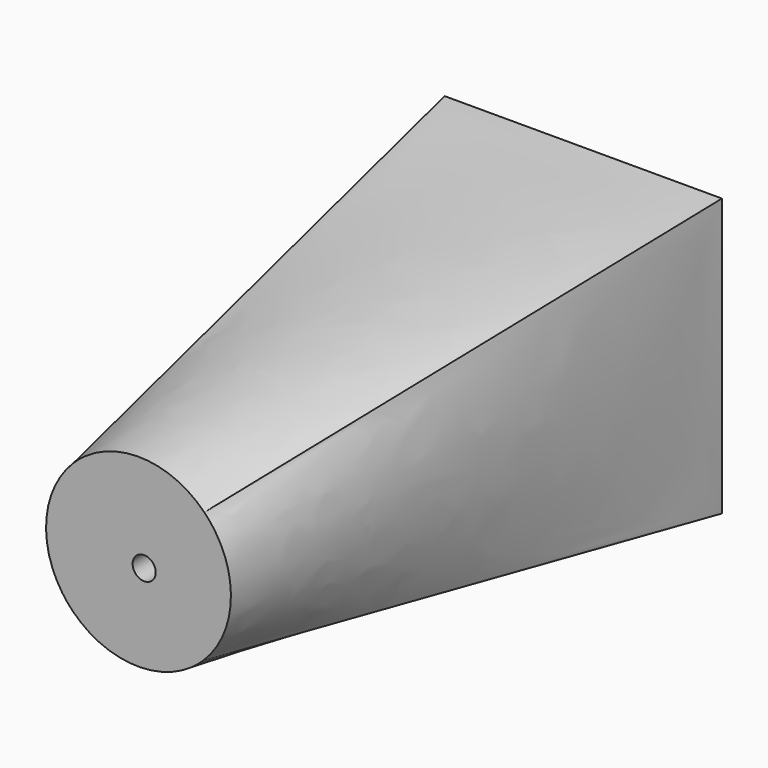
from build123d import *

# Parameters (mm, degrees)
F0_W           = 76.2
F0_H           = 76.2
F5_D           = 6.35
F5_CBORE_D     = 12.7
F5_CBORE_DEPTH = 6.35


# Not quite as in the source:
# - the arcs of a loft's sections are written as splines that run evenly, so that the points pair up as in the source's solid


with BuildPart() as f3:
    # F0 (on Front) → F3 section 0
    with BuildSketch(Plane.XZ):
        with Locations((-4.6337489039, 5.0143152279)):
            Rectangle(F0_W, F0_H)
    # F2 (on offset) → F3 section 1
    with BuildSketch(Plane.XZ.offset(152.4)):
        with BuildLine():
            add(Edge.make_bspline(
                [(-22.7580046449, 22.8249401439), (-23.9426377251, 21.6586189854), (-25.0123717458, 20.375653377), (-26.8810371807, 17.6256112299), (-27.6799223885, 16.1586026914), (-28.976175333, 13.0968432916), (-29.4735110173, 11.5021681383), (-30.1475371977, 8.2463531825), (-30.3242110272, 6.5852938864), (-30.3501079954, 3.2605425174), (-30.1993304937, 1.5969326556), (-29.5761030438, -1.6689867959), (-29.1036685059, -3.2712156294), (-27.8552669191, -6.3527957105), (-27.0793307394, -7.8320707601), (-25.2537303887, -10.6108880765), (-24.2041113593, -11.9103616316), (-23.0377902009, -13.0949947119)],
                knots=[0, 0, 0, 0, 0.125, 0.125, 0.25, 0.25, 0.375, 0.375, 0.5, 0.5, 0.625, 0.625, 0.75, 0.75, 0.875, 0.875, 1, 1, 1, 1], degree=3))
            add(Edge.make_bspline(
                [(-23.0377902009, -13.0949947119), (-21.8714690424, -14.2796277922), (-20.588503434, -15.3493618129), (-17.8384612869, -17.2180272478), (-16.3714527484, -18.0169124555), (-13.3096933486, -19.3131654), (-11.7150181953, -19.8105010844), (-8.4592032395, -20.4845272648), (-6.7981439434, -20.6612010942), (-3.4733925744, -20.6870980624), (-1.8097827126, -20.5363205608), (1.4561367389, -19.9130931108), (3.0583655724, -19.440658573), (6.1399456535, -18.1922569862), (7.6192207031, -17.4163208065), (10.3980380195, -15.5907204558), (11.6975115746, -14.5411014264), (12.8821446549, -13.3747802679)],
                knots=[0, 0, 0, 0, 0.125, 0.125, 0.25, 0.25, 0.375, 0.375, 0.5, 0.5, 0.625, 0.625, 0.75, 0.75, 0.875, 0.875, 1, 1, 1, 1], degree=3))
            add(Edge.make_bspline(
                [(12.8821446549, -13.3747802679), (14.0667777352, -12.2084591095), (15.1365117559, -10.9254935011), (17.0051771908, -8.175451354), (17.8040623985, -6.7084428155), (19.100315343, -3.6466834156), (19.5976510274, -2.0520082624), (20.2716772078, 1.2038066934), (20.4483510372, 2.8648659896), (20.4742480054, 6.1896173585), (20.3234705038, 7.8532272203), (19.7002430538, 11.1191466719), (19.227808516, 12.7213755053), (17.9794069292, 15.8029555865), (17.2034707495, 17.282230636), (15.3778703988, 20.0610479524), (14.3282513694, 21.3605215076), (13.1619302109, 22.5451545878)],
                knots=[0, 0, 0, 0, 0.125, 0.125, 0.25, 0.25, 0.375, 0.375, 0.5, 0.5, 0.625, 0.625, 0.75, 0.75, 0.875, 0.875, 1, 1, 1, 1], degree=3))
            add(Edge.make_bspline(
                [(13.1619302109, 22.5451545878), (11.9956090524, 23.7297876681), (10.7126434441, 24.7995216888), (7.962601297, 26.6681871237), (6.4955927584, 27.4670723315), (3.4338333586, 28.763325276), (1.8391582054, 29.2606609603), (-1.4166567504, 29.9346871407), (-3.0777160466, 30.1113609702), (-6.4024674155, 30.1372579384), (-8.0660772773, 29.9864804367), (-11.3319967289, 29.3632529868), (-12.9342255623, 28.8908184489), (-16.0158056435, 27.6424168621), (-17.495080693, 26.8664806824), (-20.2738980095, 25.0408803317), (-21.5733715646, 23.9912613023), (-22.7580046449, 22.8249401439)],
                knots=[0, 0, 0, 0, 0.125, 0.125, 0.25, 0.25, 0.375, 0.375, 0.5, 0.5, 0.625, 0.625, 0.75, 0.75, 0.875, 0.875, 1, 1, 1, 1], degree=3))
        make_face()
    loft(ruled=True)

    # F5 (through all)
    with Locations(Plane(origin=(0, 0, 0), x_dir=(-1, 0, 0), z_dir=(0, 1, 0))):
        with Locations((3.3759707585, 3.656350309)):
            CounterBoreHole(F5_D / 2, F5_CBORE_D / 2, F5_CBORE_DEPTH)


solid = f3.part
